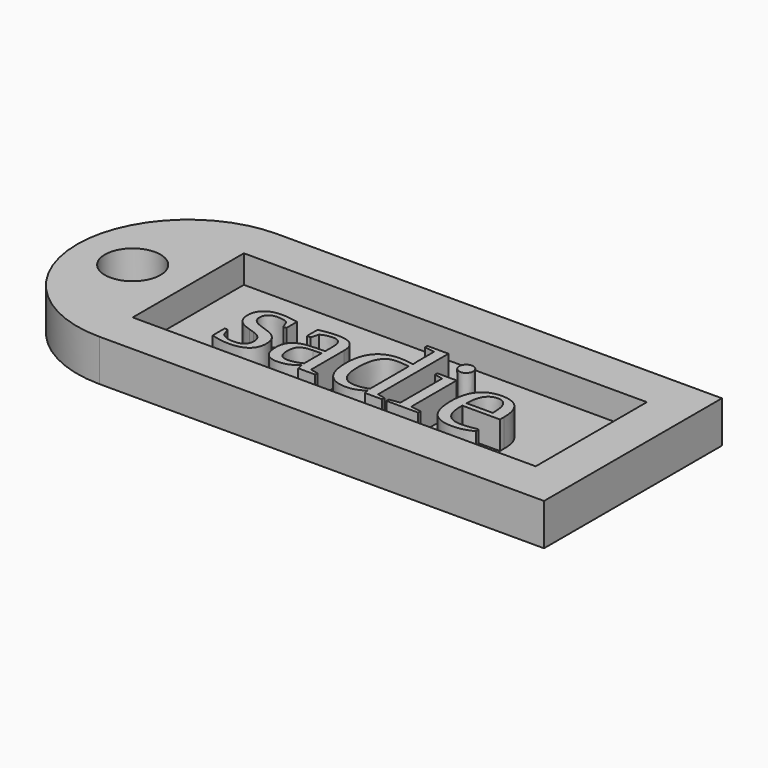
from build123d import *

# Parameters (mm, degrees)
F1_DEPTH     = 3.81
F2_W         = 36.83
F2_H         = 12.7
F3_DEPTH     = 2.54
F4_R         = 2.54
F5_DEPTH     = 25.4
F6_TEXT_SIZE = 12.1959636882
F7_DEPTH     = 2.54


# Not quite as in the source:
# - Text() gives the source's letters only with a copy of the font that has no kerning and outlines rounded to 1/6400 em; it was checked with that copy


with BuildPart() as f1:
    # F0 (on Top) → F1 (new body)
    with BuildSketch(Plane.XY):
        with BuildLine():
            ThreePointArc((-32.4928554767, 38.1459156051), (-29.5170603735, 30.9617107083), (-22.3328554767, 27.9859156051))
            Line((-22.3328554767, 27.9859156051), (18.3071445233, 27.9859156051))
            Line((18.3071445233, 27.9859156051), (18.3071445233, 48.3059156051))
            Line((18.3071445233, 48.3059156051), (-22.3328554767, 48.3059156051))
            ThreePointArc((-22.3328554767, 48.3059156051), (-29.5170603735, 45.330120502), (-32.4928554767, 38.1459156051))
        make_face()
    extrude(amount=F1_DEPTH)

    # F2 (on face) → F3 (cut)
    with BuildSketch(Plane.XY.offset(3.81)):
        with Locations((-3.9178554767, 38.1459156051)):
            Rectangle(F2_W, F2_H)
    extrude(amount=-F3_DEPTH, mode=Mode.SUBTRACT)

    # F4 (on face) → F5 (cut)
    with BuildSketch(Plane.XY.offset(3.81)):
        with Locations((-27.4128554767, 38.1459156051)):
            Circle(F4_R)
    extrude(amount=-F5_DEPTH, mode=Mode.SUBTRACT)

    # F6 (on face) → F7 (join)
    with BuildSketch(Plane.XY.offset(1.27)):
        with Locations((-16.6550166482, 33.035718249)):
            Text('sadie', F6_TEXT_SIZE, font='Tinos', text_align=(TextAlign.LEFT, TextAlign.BOTTOM))
    extrude(amount=F7_DEPTH)


solid = f1.part
